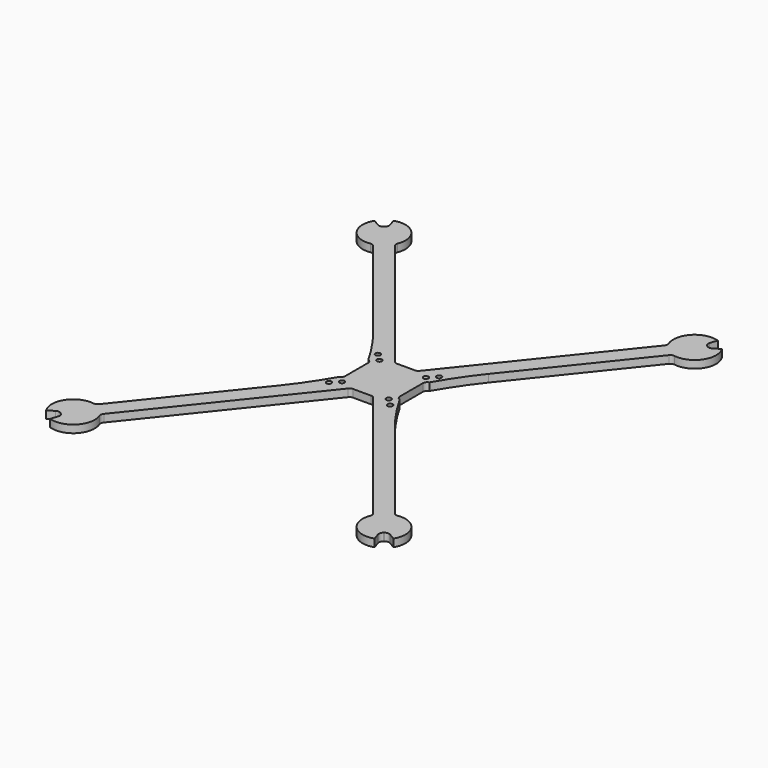
from build123d import *

# Parameters (mm, degrees)
F0_R        = 1.65
F1_DEPTH    = 5
F2_T1_DEPTH = 5
F3_T1_DEPTH = 5


# Not quite as in the source:
# - a fillet or chamfer that OpenCascade refuses, or shapes differently, is made with other operations: its cross-section is extruded or revolved along the edge and cut away or added


with BuildPart() as f1:
    # F0 (on Top) → F1 (new body)
    with BuildSketch(Plane.XY):
        Polygon((7.0434366612, 0), (14.0868733224, 0), (17.9254915565, 0), (17.9254915565, 12.1765555814), (17.9254915565, 13.6025686192), align=None)
        Polygon((0, 0), (7.0434366612, 0), (17.9254915565, 13.6025686192), (17.9254915565, 17.9254915565), (7.296956584, 17.9254915565), (0, 8.8042958265), align=None)
        with Locations((15.25, 15.25)):
            Circle(F0_R, mode=Mode.SUBTRACT)
        with BuildLine():
            Line((17.9254915565, 17.9254915565), (17.9254915565, 13.6025686192))
            Line((17.9254915565, 13.6025686192), (17.9254915565, 12.1765555814))
            Line((17.9254915565, 12.1765555814), (20, 12.1765555814))
            Line((20, 12.1765555814), (23.3218736491, 20.3480462349))
            Line((23.3218736491, 20.3480462349), (97.8522087861, 113.5109651562))
            ThreePointArc((97.8522087861, 113.5109651562), (92.8542693342, 116.0678366678), (89.2626518823, 120.3826106793))
            Line((89.2626518823, 120.3826106793), (7.296956584, 17.9254915565))
            Line((7.296956584, 17.9254915565), (17.9254915565, 17.9254915565))
        make_face()
        with Locations((20, 20)):
            Circle(F0_R, mode=Mode.SUBTRACT)
        Polygon((0, 17.9254915565), (0, 8.8042958265), (7.296956584, 17.9254915565), align=None)
        with BuildLine():
            ThreePointArc((106.0792785003, 140.2640892683), (90.9109583101, 136.0412602966), (89.2626518823, 120.3826106793))
            ThreePointArc((89.2626518823, 120.3826106793), (92.8542693342, 116.0678366678), (97.8522087861, 113.5109651562))
            ThreePointArc((97.8522087861, 113.5109651562), (112.7671167579, 118.5563335383), (113.5573186397, 134.2816571567))
            Line((113.5573186397, 134.2816571567), (107.5786593199, 130.6408285784))
            Line((107.5786593199, 130.6408285784), (103.8396392501, 133.6320446341))
            Line((103.8396392501, 133.6320446341), (106.0792785003, 140.2640892683))
        make_face()
    extrude(amount=F1_DEPTH)

    # F2: fillet of radius 3 on 6 edges, made by hand

    # F2_s2 → F2_t1 (join)
    with BuildSketch(Plane.XY):
        with BuildLine():
            ThreePointArc((8.1976884699, 19.0514064139), (7.1546482331, 18.2215818476), (5.8550820416, 17.9254915565))
            Line((5.8550820416, 17.9254915565), (7.296956584, 17.9254915565))
            Line((7.296956584, 17.9254915565), (8.1976884699, 19.0514064139))
        make_face()
        with BuildLine():
            ThreePointArc((17.9254915565, 9.3228798152), (18.4989225106, 11.0868987111), (20, 12.1765555814))
            Line((20, 12.1765555814), (17.9254915565, 12.1765555814))
            Line((17.9254915565, 12.1765555814), (17.9254915565, 9.3228798152))
        make_face()
        with BuildLine():
            ThreePointArc((96.6977481783, 112.0678893964), (97.9486405, 112.9881128103), (99.4920567349, 113.1596035031))
            ThreePointArc((99.4920567349, 113.1596035031), (98.6668668075, 113.3107074808), (97.8522087861, 113.5109651562))
            Line((97.8522087861, 113.5109651562), (96.6977481783, 112.0678893964))
        make_face()
        with BuildLine():
            ThreePointArc((88.5598934027, 121.9053341689), (88.7313840955, 120.361917934), (88.1081912745, 118.9395349195))
            Line((88.1081912745, 118.9395349195), (89.2626518823, 120.3826106793))
            ThreePointArc((89.2626518823, 120.3826106793), (88.8884511699, 121.1334399909), (88.5598934027, 121.9053341689))
        make_face()
        with BuildLine():
            ThreePointArc((105.4799499303, 132.31979609), (104.4752105502, 133.8183827512), (104.5117302298, 135.6222479112))
            Line((104.5117302298, 135.6222479112), (103.8396392501, 133.6320446341))
            Line((103.8396392501, 133.6320446341), (105.4799499303, 132.31979609))
        make_face()
        with BuildLine():
            ThreePointArc((109.3727888874, 131.7334009852), (107.6209369535, 131.3018016285), (105.9383486397, 131.9530771225))
            Line((105.9383486397, 131.9530771225), (107.5786593199, 130.6408285784))
            Line((107.5786593199, 130.6408285784), (109.3727888874, 131.7334009852))
        make_face()
    extrude(amount=F2_T1_DEPTH)

    # F3: fillet of radius 199.9181440352 on 1 edges, made by hand

    # F3_s2 → F3_t1 (join)
    with BuildSketch(Plane.XY):
        with BuildLine():
            ThreePointArc((20, 12.1765555814), (28.3645778619, 25.6450570093), (37.770134119, 38.4083718223))
            Line((37.770134119, 38.4083718223), (23.3218736491, 20.3480462349))
            Line((23.3218736491, 20.3480462349), (20, 12.1765555814))
        make_face()
    extrude(amount=F3_T1_DEPTH)

    # F4: F1 across plane


with BuildPart() as f1_1:
    add(f1.part)
    add(f1.part.mirror(Plane.YZ))

    # F5: F1 across plane


with BuildPart() as f1_2:
    add(f1_1.part)
    add(f1_1.part.mirror(Plane.XZ))


solid = f1_2.part
